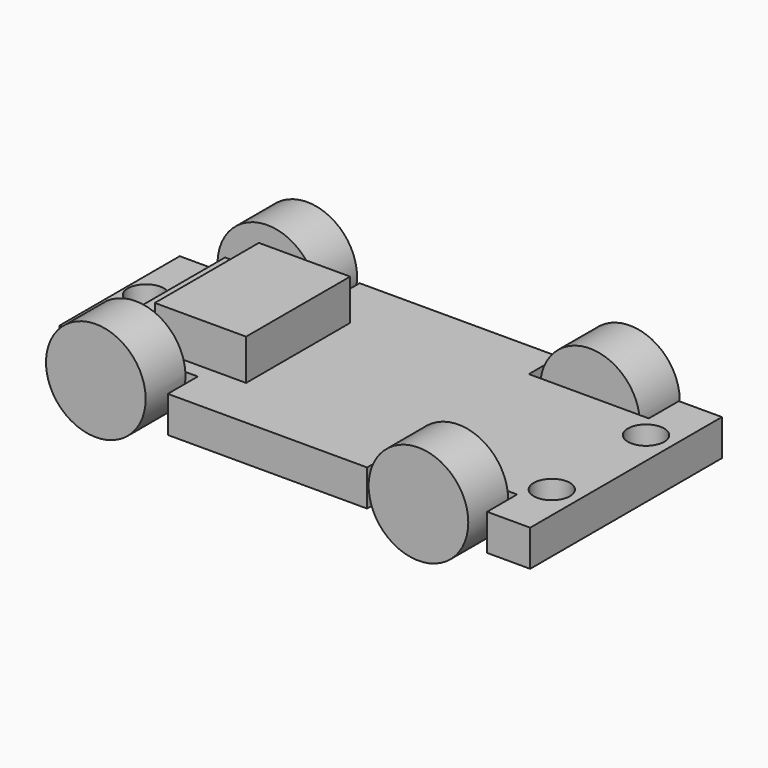
from build123d import *

# Parameters (mm, degrees)
F0_R      = 4
F1_DEPTH  = 8
F2_W      = 10
F2_H      = 33.13
F3_DEPTH  = 3
F4_R      = 1.5
F5_DEPTH  = 26
F6_W      = 20.15
F6_H      = 28.71
F7_DEPTH  = 9
F8_R      = 11
F9_DEPTH  = 11
F10_R     = 1.25
F11_DEPTH = 47.351
F12_R     = 11
F13_DEPTH = 11


# Not quite as in the source:
# - a pattern or mirror of a feature is missing from the dataset's text; its kind, count and spacing are read off the source's solid


with BuildPart() as f1:
    # F0 (on Top) → F1 (new body)
    with BuildSketch(Plane.XY):
        Polygon((55.25, -26.455), (55.25, 26.455), (45.74, 26.455), (45.74, 18.175), (19.25, 18.175), (19.25, 26.455), (-24.73, 26.455), (-24.73, 14.955), (-55.25, 14.955), (-55.25, -18.175), (-24.75, -18.175), (-24.75, -26.455), (19.25, -26.455), (19.25, -18.175), (45.74, -18.175), (45.74, -26.455), align=None)
        with Locations((49.26, -13)):
            Circle(F0_R, mode=Mode.SUBTRACT)
        with Locations((-50.74, 0)):
            Circle(F0_R, mode=Mode.SUBTRACT)
        with Locations((49.26, 13)):
            Circle(F0_R, mode=Mode.SUBTRACT)
    extrude(amount=F1_DEPTH)

    # F2 (on face) → F3 (join)
    with BuildSketch(Plane.XY.offset(8)):
        with Locations((-40.25, -1.61)):
            Rectangle(F2_W, F2_H)
    extrude(amount=F3_DEPTH)

    # F4 (on Front) → F5 (join, symmetric)
    with BuildSketch(Plane.XZ):
        with Locations((-38.47, 7.2)):
            Circle(F4_R)
    extrude(amount=F5_DEPTH, both=True)

    # F6 (on face) → F7 (join)
    with BuildSketch(Plane.XY.offset(8)):
        with Locations((-26.825, -0.5)):
            Rectangle(F6_W, F6_H)
    extrude(amount=F7_DEPTH)

    # F8 (on face) → F9 (join)
    with BuildSketch(Plane.XZ.offset(18.175)):
        with Locations((-38.47, 7.2)):
            Circle(F8_R)
    f9 = extrude(amount=F9_DEPTH)

    # F9_copies: F9 across plane
    add(f9.mirror(Plane.ZX))

    # F10 (on face) → F11 (cut, through all)
    with BuildSketch(Plane.XZ.offset(18.175)):
        with Locations((32.76, 6.375)):
            Circle(F10_R)
    extrude(amount=-F11_DEPTH, mode=Mode.SUBTRACT)

    # F12 (on face) → F13 (join)
    with BuildSketch(Plane.XZ.offset(18.175)):
        with Locations((32.76, 6.375)):
            Circle(F12_R)
    f13 = extrude(amount=F13_DEPTH)

    # F13_copies: F13 across plane
    add(f13.mirror(Plane.ZX))


solid = f1.part
